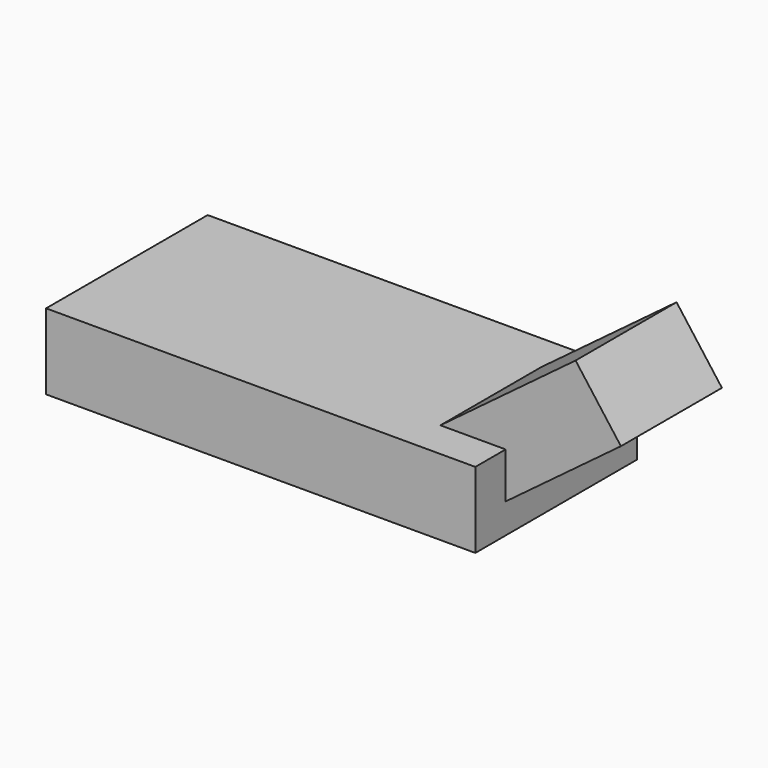
from build123d import *

# Parameters (mm, degrees)
F0_W     = 170
F0_H     = 80
F1_DEPTH = 30
F3_DEPTH = 61.7
F4_DEPTH = 14.1
F7_DEPTH = 3.3
F8_DEPTH = 0.9


with BuildPart() as f1:
    # F0 (on Top) → F1 (new body)
    with BuildSketch(Plane.XY):
        Rectangle(F0_W, F0_H)
    extrude(amount=F1_DEPTH)


with BuildPart() as f3:
    # F2 (on face) → F3 (new body)
    with BuildSketch(Plane.XZ.offset(40)):
        Polygon((112.6936972141, 69.9990615249), (59.1574877457, 30), (85, 30), (85, 11.8593943491), (130.649682243, 45.9661132737), align=None)
    extrude(amount=-F3_DEPTH)

    # F4 (cut): a face of the model
    f4_faces = [f3.faces().sort_by_distance(p)[0] for p in [
        (99.5026263907, -40, 42.0152443758),
    ]]
    extrude(f4_faces, amount=-F4_DEPTH, mode=Mode.SUBTRACT)

    # F7 (add, through all): a face of the model
    f7_faces = [f3.faces().sort_by_distance(p)[0] for p in [
        (99.5026263907, 21.7, 42.0152443758),
    ]]
    extrude(f7_faces, amount=F7_DEPTH)

    # F8 (cut, through all): a face of the model
    f8_faces = [f3.faces().sort_by_distance(p)[0] for p in [
        (99.5026263907, -25.9, 42.0152443758),
    ]]
    extrude(f8_faces, amount=-F8_DEPTH, mode=Mode.SUBTRACT)


solid = Compound([f1.part, f3.part])
